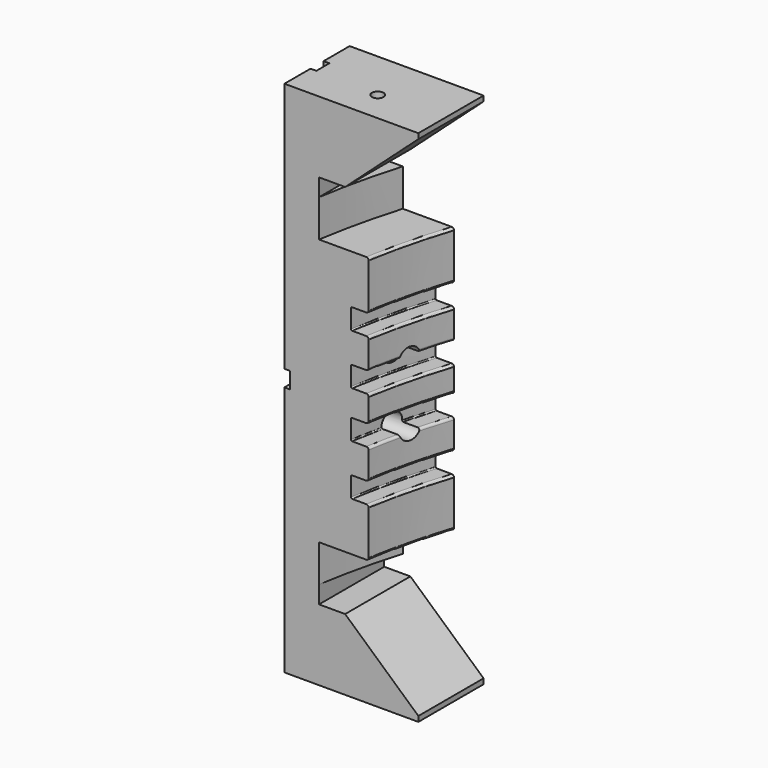
from build123d import *

# Parameters (mm, degrees)
F4_DEPTH  = 292.8
F6_DEPTH  = 292.8
F8_DEPTH  = 70
F10_DEPTH = 5
F11_R     = 5.5
F12_DEPTH = 591
F14_R     = 8.5
F15_DEPTH = 587
F16_R     = 5
F17_DEPTH = 18
F18_R     = 5
F19_DEPTH = 18


# Not quite as in the source:
# - an extrude ends at something that could not be found from the text; its depth is read off the source's solid


with BuildPart() as f2:
    # F2: sweep along a path in F0
    with BuildLine(Plane.XY) as f2_path:
        ThreePointArc((-433.0127018922, 250), (-482.9629131445, 129.4095225513), (-500, 0))
    # F1 (on Front) → F2 (sweep)
    with BuildSketch(Plane.XZ):
        with BuildLine():
            Line((-500, -9.2), (-500, 0))
            Line((-500, 0), (-500, 9.2))
            ThreePointArc((-500, 9.2), (-500.5857864376, 10.6142135624), (-502, 11.2))
            Line((-502, 11.2), (-514, 11.2))
            ThreePointArc((-514, 11.2), (-514.7071067812, 11.4928932188), (-515, 12.2))
            Line((-515, 12.2), (-515, 27.9))
            ThreePointArc((-515, 27.9), (-514.7071067812, 28.6071067812), (-514, 28.9))
            Line((-514, 28.9), (-502, 28.9))
            ThreePointArc((-502, 28.9), (-500.5857864376, 29.4857864376), (-500, 30.9))
            Line((-500, 30.9), (-500, 52.56))
            ThreePointArc((-500, 52.56), (-500.6150757595, 54.0449242405), (-502.1, 54.66))
            Line((-502.1, 54.66), (-514, 54.66))
            ThreePointArc((-514, 54.66), (-514.7071067812, 54.9528932188), (-515, 55.66))
            Line((-515, 55.66), (-515, 71.44))
            ThreePointArc((-515, 71.44), (-514.7071067812, 72.1471067812), (-514, 72.44))
            Line((-514, 72.44), (-502, 72.44))
            ThreePointArc((-502, 72.44), (-500.5857864376, 73.0257864376), (-500, 74.44))
            Line((-500, 74.44), (-500, 112.4))
            ThreePointArc((-500, 112.4), (-500.5857864376, 113.8142135624), (-502, 114.4))
            Line((-502, 114.4), (-542, 114.4))
            Line((-542, 114.4), (-542, 146.4))
            Line((-542, 146.4), (-565, 146.4))
            Line((-565, 146.4), (-565, 0))
            Line((-565, 0), (-565, -146.4))
            Line((-565, -146.4), (-542, -146.4))
            Line((-542, -146.4), (-542, -114.4))
            Line((-542, -114.4), (-502, -114.4))
            ThreePointArc((-502, -114.4), (-500.5857864376, -113.8142135624), (-500, -112.4))
            Line((-500, -112.4), (-500, -74.44))
            ThreePointArc((-500, -74.44), (-500.5857864376, -73.0257864376), (-502, -72.44))
            Line((-502, -72.44), (-514, -72.44))
            ThreePointArc((-514, -72.44), (-514.7071067812, -72.1471067812), (-515, -71.44))
            Line((-515, -71.44), (-515, -55.66))
            ThreePointArc((-515, -55.66), (-514.7071067812, -54.9528932188), (-514, -54.66))
            Line((-514, -54.66), (-502.1, -54.66))
            ThreePointArc((-502.1, -54.66), (-500.6150757595, -54.0449242405), (-500, -52.56))
            Line((-500, -52.56), (-500, -30.9))
            ThreePointArc((-500, -30.9), (-500.5857864376, -29.4857864376), (-502, -28.9))
            Line((-502, -28.9), (-514, -28.9))
            ThreePointArc((-514, -28.9), (-514.7071067812, -28.6071067812), (-515, -27.9))
            Line((-515, -27.9), (-515, -12.2))
            ThreePointArc((-515, -12.2), (-514.7071067812, -11.4928932188), (-514, -11.2))
            Line((-514, -11.2), (-502, -11.2))
            ThreePointArc((-502, -11.2), (-500.5857864376, -10.6142135624), (-500, -9.2))
        make_face()
    sweep(path=f2_path.line)

    # F3 (on face) → F4 (join, through all)
    with BuildSketch(Plane.XY.offset(146.4)):
        with BuildLine():
            Line((-565, 85), (-558.5696017508, 85))
            ThreePointArc((-558.5696017508, 85), (-552.0569591168, 120.2418974016), (-543.3231082882, 155))
            Line((-543.3231082882, 155), (-565, 155))
            Line((-565, 155), (-565, 85))
        make_face()
    extrude(amount=-F4_DEPTH)

    # F5 (on face) → F6 (cut, through all)
    with BuildSketch(Plane.XY.offset(146.4)):
        with BuildLine():
            Line((-492.7220311697, 85), (-535.2933775043, 85))
            ThreePointArc((-535.2933775043, 85), (-540.3207429885, 42.6320852918), (-542, 0))
            Line((-542, 0), (-500, 0))
            ThreePointArc((-500, 0), (-498.1771851384, 42.6555061812), (-492.7220311697, 85))
        make_face()
        with BuildLine():
            ThreePointArc((-542, 0), (-540.3207429885, 42.6320852918), (-535.2933775043, 85))
            Line((-535.2933775043, 85), (-558.5696017508, 85))
            ThreePointArc((-558.5696017508, 85), (-563.3901068483, 42.6214441967), (-565, 0))
            Line((-565, 0), (-542, 0))
        make_face()
        with BuildLine():
            ThreePointArc((-489.3043531382, 282.5), (-520.2344961871, 220.4111362363), (-543.3231082882, 155))
            Line((-543.3231082882, 155), (-519.3640341803, 155))
            ThreePointArc((-519.3640341803, 155), (-497.765550484, 214.4608513257), (-469.3857688512, 271))
            Line((-469.3857688512, 271), (-489.3043531382, 282.5))
        make_face()
        with BuildLine():
            ThreePointArc((-469.3857688512, 271), (-497.765550484, 214.4608513257), (-519.3640341803, 155))
            Line((-519.3640341803, 155), (-475.3682782854, 155))
            ThreePointArc((-475.3682782854, 155), (-456.6675500702, 203.604392666), (-433.0127018922, 250))
            Line((-433.0127018922, 250), (-469.3857688512, 271))
        make_face()
    extrude(amount=-F6_DEPTH, mode=Mode.SUBTRACT)

    # F7 (on face) → F8 (join, through all)
    with BuildSketch(Plane.XZ.offset(-85)):
        Polygon((-535.2933775043, -146.4), (-565, -146.4), (-565, -222.5), (-450, -222.5), (-450, -217.9979797785), (-512.8584246561, -161.4), (-535.2933775043, -161.4), align=None)
        Polygon((-565, 222.5), (-565, 146.4), (-535.2933775043, 146.4), (-535.2933775043, 161.4), (-512.8584246561, 161.4), (-450, 217.9979797785), (-450, 222.5), align=None)
    extrude(amount=-F8_DEPTH)

    # F9 (on face) → F10 (cut)
    with BuildSketch(Plane(origin=(-565, 0, 0), x_dir=(0, -1, 0), z_dir=(-1, 0, 0))):
        Polygon((-113, 222.5), (-127, 222.5), (-127, 7), (-155, 7), (-155, -7), (-127, -7), (-127, -222.5), (-113, -222.5), (-113, -7), (-85, -7), (-85, 7), (-113, 7), align=None)
    extrude(amount=-F10_DEPTH, mode=Mode.SUBTRACT)

    # F11 (on face) → F12 (cut, through all)
    with BuildSketch(Plane(origin=(-560, 0, 0), x_dir=(0, -1, 0), z_dir=(-1, 0, 0))):
        with Locations((-120, 27)):
            Circle(F11_R)
        with Locations((-120, -27)):
            Circle(F11_R)
    extrude(amount=-F12_DEPTH, mode=Mode.SUBTRACT)

    # F14 (on offset) → F15 (cut, through all)
    with BuildSketch(Plane.YZ.offset(-513.77)):
        with Locations((120, 27)):
            Circle(F14_R)
        with Locations((120, -27)):
            Circle(F14_R)
    extrude(amount=F15_DEPTH, mode=Mode.SUBTRACT)

    # F16 (on face) → F17 (cut)
    with BuildSketch(Plane.XY.offset(222.5)):
        with Locations((-506, 111.4)):
            Circle(F16_R)
    extrude(amount=-F17_DEPTH, mode=Mode.SUBTRACT)

    # F18 (on face) → F19 (cut)
    with BuildSketch(Plane(origin=(0, 0, -222.5), x_dir=(1, 0, 0), z_dir=(0, 0, -1))):
        with Locations((-506, -128.6)):
            Circle(F18_R)
    extrude(amount=-F19_DEPTH, mode=Mode.SUBTRACT)


solid = f2.part
